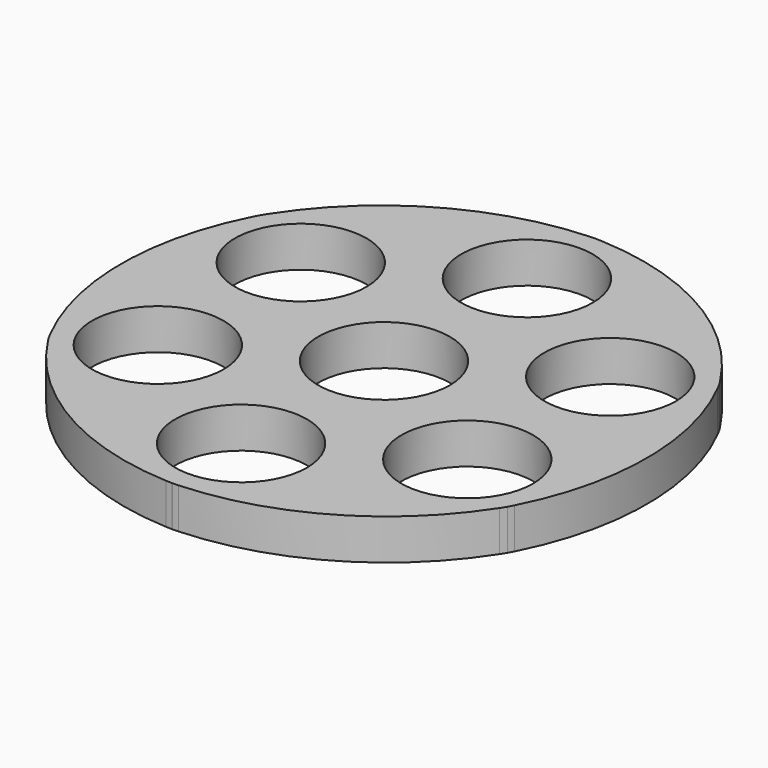
from build123d import *

# Parameters (mm, degrees)
F0_R     = 10.6
F1_DEPTH = 5
F0_R_2   = 8.1
F2_DEPTH = 5


# Not quite as in the source:
# - ends of sketch curves that miss each other by under 0.0002 mm in the source are joined


with BuildPart() as f1:
    # F0 (on Top) → F1 (new body)
    with BuildSketch(Plane.XY):
        with BuildLine():
            ThreePointArc((27.8263414504, 16.9481692723), (16.199467196, 28.0319950031), (0.7904601582, 32.5704859273))
            ThreePointArc((0.7904601582, 32.5704859273), (7.7697772708, 29.2104480555), (10.6, 22))
            ThreePointArc((10.6, 22), (-7.2200130901, 14.2391101684), (-0.7644171658, 32.5724011651))
            ThreePointArc((-0.7644171658, 32.5724011651), (-16.1766867062, 28.0451473253), (-27.8116156006, 16.9698365243))
            ThreePointArc((-27.8116156006, 16.9698365243), (-15.9289393792, 21.1293147465), (-8.4525595083, 11.0000009845))
            ThreePointArc((-8.4525595083, 11.0000009845), (-21.4248089079, 0.6688619967), (-28.5907543736, 15.6241591469))
            ThreePointArc((-28.5907543736, 15.6241591469), (-32.3761533963, 0.0131339969), (-28.6021197402, -15.6006426749))
            ThreePointArc((-28.6021197402, -15.6006426749), (-21.4120811641, -0.665945501), (-8.4525606734, -10.9999990645))
            ThreePointArc((-8.4525606734, -10.9999990645), (-15.9414195658, -21.1331526215), (-27.8262967127, -16.9482387968))
            ThreePointArc((-27.8262967127, -16.9482387968), (-16.1994359735, -28.0320130446), (-0.7904706999, -32.5704854113))
            ThreePointArc((-0.7904706999, -32.5704854113), (-7.2104473679, -14.2302200266), (10.5999976698, -22.0000000981))
            ThreePointArc((10.5999976698, -22.0000000981), (7.7608872989, -29.2200134059), (0.7644142424, -32.5724013061))
            ThreePointArc((0.7644142424, -32.5724013061), (16.17671692, -28.045129896), (27.8116549786, -16.9697754267))
            ThreePointArc((27.8116549786, -16.9697754267), (8.9232325044, -7.8764163379), (29.652557178, -11.0000010826))
            ThreePointArc((29.652557178, -11.0000010826), (29.3836867135, -13.3722916469), (28.5907151929, -15.6242352553))
            ThreePointArc((28.5907151929, -15.6242352553), (32.3761533958, -0.0131351765), (28.6020816932, 15.6007167134))
            ThreePointArc((28.6020816932, 15.6007167134), (29.3866027477, 13.3595595706), (29.6525583432, 10.9999989665))
            ThreePointArc((29.6525583432, 10.9999989665), (8.9193924771, 7.8888979505), (27.8263414504, 16.9481692723))
        make_face()
        Circle(F0_R, mode=Mode.SUBTRACT)
    extrude(amount=F1_DEPTH)

    # F0 (on Top) → F2 (join)
    with BuildSketch(Plane.XY):
        with BuildLine():
            ThreePointArc((28.2460392226, -16.2763527502), (28.4201387166, -15.9512250463), (28.5907151929, -15.6242352553))
            ThreePointArc((28.5907151929, -15.6242352553), (29.3836867135, -13.3722916469), (29.652557178, -11.0000010826))
            ThreePointArc((29.652557178, -11.0000010826), (8.9232325044, -7.8764163379), (27.8116549786, -16.9697754267))
            ThreePointArc((27.8116549786, -16.9697754267), (28.023981709, -16.6361065668), (28.2324281634, -16.3))
            ThreePointArc((28.2324281634, -16.3), (28.2392409163, -16.2881805324), (28.2460392226, -16.2763527502))
        make_face()
        with Locations((19.052557178, -11.0000010826)):
            Circle(F0_R_2, mode=Mode.SUBTRACT)
        with BuildLine():
            ThreePointArc((28.2187545739, 16.3236111479), (28.0242350806, 16.636950204), (27.8263414504, 16.9481692723))
            ThreePointArc((27.8263414504, 16.9481692723), (8.9193924771, 7.8888979505), (29.6525583432, 10.9999989665))
            ThreePointArc((29.6525583432, 10.9999989665), (29.3866027477, 13.3595595706), (28.6020816932, 15.6007167134))
            ThreePointArc((28.6020816932, 15.6007167134), (28.4192805282, 15.9514291247), (28.2324281634, 16.3))
            ThreePointArc((28.2324281634, 16.3), (28.2255985395, 16.3118097271), (28.2187545739, 16.3236111479))
        make_face()
        with Locations((19.0525583432, 10.9999989665)):
            Circle(F0_R_2, mode=Mode.SUBTRACT)
        with BuildLine():
            ThreePointArc((0.0272846487, -32.5999638982), (0.3959239022, -32.5881738584), (0.7644142424, -32.5724013061))
            ThreePointArc((0.7644142424, -32.5724013061), (7.7608872989, -29.2200134059), (10.5999976698, -22.0000000981))
            ThreePointArc((10.5999976698, -22.0000000981), (-7.2104473679, -14.2302200266), (-0.7904706999, -32.5704854113))
            ThreePointArc((-0.7904706999, -32.5704854113), (-0.3953208493, -32.5875325821), (0, -32.6))
            ThreePointArc((0, -32.6), (0.013642337, -32.5999913161), (0.0272846487, -32.5999638982))
        make_face()
        with Locations((-2.3302e-06, -22.0000000981)):
            Circle(F0_R_2, mode=Mode.SUBTRACT)
        Circle(F0_R)
        Circle(F0_R_2, mode=Mode.SUBTRACT)
        with BuildLine():
            ThreePointArc((-8.4525606734, -10.9999990645), (-21.4120811641, -0.665945501), (-28.6021197402, -15.6006426749))
            ThreePointArc((-28.6021197402, -15.6006426749), (-28.4192999794, -15.9513923284), (-28.2324281634, -16.3))
            ThreePointArc((-28.2324281634, -16.3), (-28.2256003271, -16.3118107622), (-28.218756359, -16.3236121847))
            ThreePointArc((-28.218756359, -16.3236121847), (-28.0242130887, -16.6369852059), (-27.8262967127, -16.9482387968))
            ThreePointArc((-27.8262967127, -16.9482387968), (-15.9414195658, -21.1331526215), (-8.4525606734, -10.9999990645))
        make_face()
        with Locations((-19.0525606734, -10.9999990645)):
            Circle(F0_R_2, mode=Mode.SUBTRACT)
        with BuildLine():
            ThreePointArc((-8.4525595083, 11.0000009845), (-15.9289393792, 21.1293147465), (-27.8116156006, 16.9698365243))
            ThreePointArc((-27.8116156006, 16.9698365243), (-28.0239623753, 16.6361373416), (-28.2324281634, 16.3))
            ThreePointArc((-28.2324281634, 16.3), (-28.2392426242, 16.2881815155), (-28.2460409731, 16.2763537548))
            ThreePointArc((-28.2460409731, 16.2763537548), (-28.420158717, 15.951187206), (-28.5907543736, 15.6241591469))
            ThreePointArc((-28.5907543736, 15.6241591469), (-21.4248089079, 0.6688619967), (-8.4525595083, 11.0000009845))
        make_face()
        with Locations((-19.0525595083, 11.0000009845)):
            Circle(F0_R_2, mode=Mode.SUBTRACT)
        with BuildLine():
            ThreePointArc((0.7904601582, 32.5704859273), (0.3953155758, 32.587532779), (0, 32.6))
            ThreePointArc((0, 32.6), (-0.0136423369, 32.5999912211), (-0.0272846512, 32.5999648843))
            ThreePointArc((-0.0272846512, 32.5999648843), (-0.3959253645, 32.5881738038), (-0.7644171658, 32.5724011651))
            ThreePointArc((-0.7644171658, 32.5724011651), (-7.2200130901, 14.2391101684), (10.6, 22))
            ThreePointArc((10.6, 22), (7.7697772708, 29.2104480555), (0.7904601582, 32.5704859273))
        make_face()
        with Locations((0, 22)):
            Circle(F0_R_2, mode=Mode.SUBTRACT)
    extrude(amount=F2_DEPTH)


solid = f1.part
